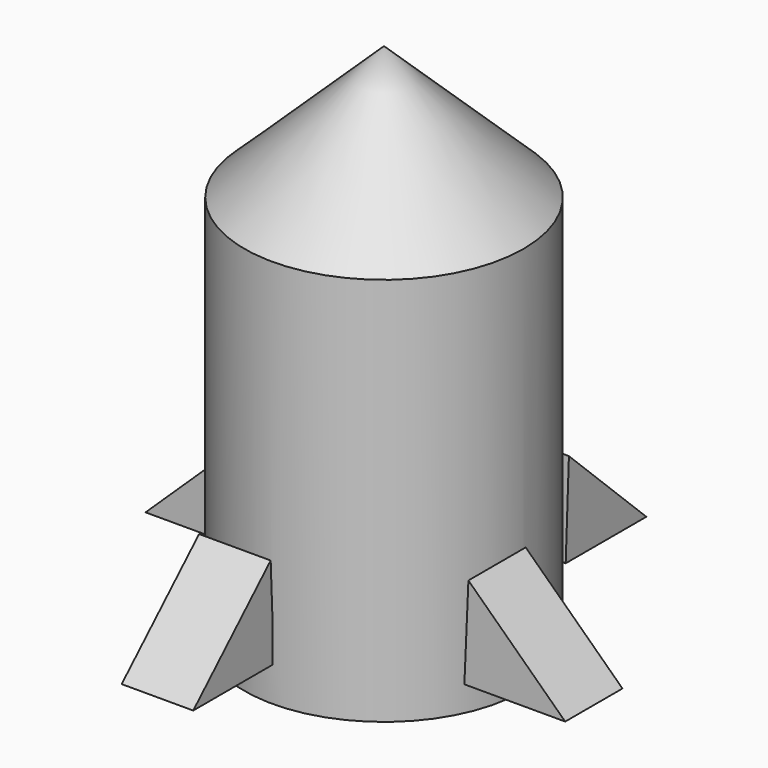
from build123d import *

# Parameters (mm, degrees)
F3_DEPTH        = 10
F3_COPIES_COUNT = 4


# Not quite as in the source:
# - a pattern or mirror of a feature is missing from the dataset's text; its kind, count and spacing are read off the source's solid


with BuildPart() as f1:
    # F0 (on Front) → F1 (revolve)
    with BuildSketch(Plane.XZ):
        Polygon((19.5114035159, 23.0333190411), (0, 41.6290275753), (0, -31.3450358808), (19.5114035159, -31.3450358808), align=None)
    revolve(axis=Axis((0, 0, 5.1419958472), (0, 0, -1)))

    # F2 (on Right) → F3 (join)
    with BuildSketch(Plane.YZ):
        Polygon((-19.2296542227, -26.5552345663), (-19.7931565344, -13.5945891961), (-33.3173125982, -26.5552345663), align=None)
    f3 = extrude(amount=-F3_DEPTH)

    # F3_copies: F3 ×4 about axis
    f3_copies_axis = Axis((0, 0, 0), (0, 0, 1))
    for i in range(1, F3_COPIES_COUNT):
        add(f3.rotate(f3_copies_axis, i * 360 / F3_COPIES_COUNT))


solid = f1.part
